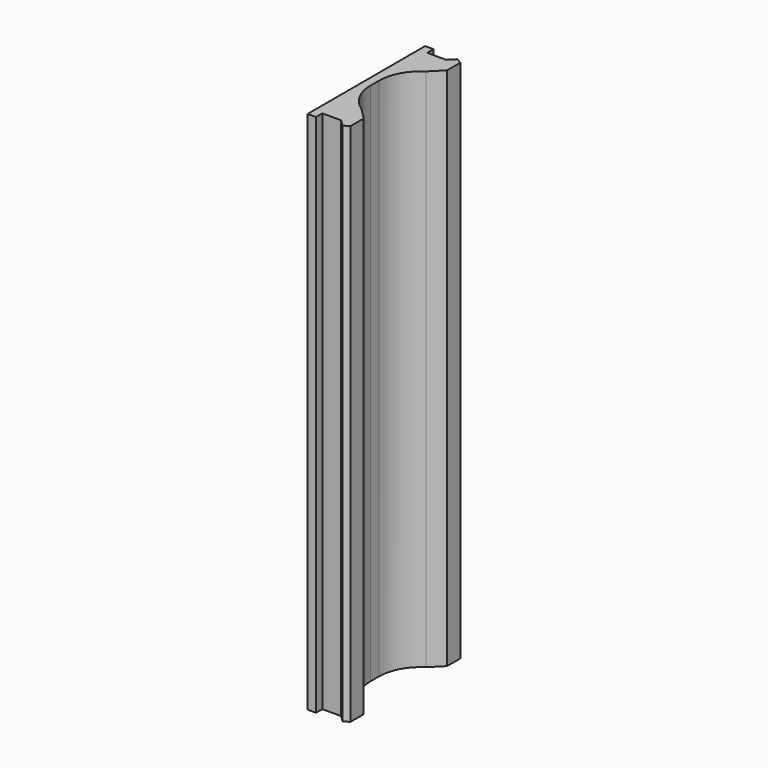
from build123d import *

# Parameters (mm, degrees)
F1_DEPTH    = 25
F2_T1_DEPTH = 25


# Not quite as in the source:
# - a fillet or chamfer that OpenCascade refuses, or shapes differently, is made with other operations: its cross-section is extruded or revolved along the edge and cut away or added


with BuildPart() as f1:
    # F0 (on Top) → F1 (new body)
    with BuildSketch(Plane.XY):
        Polygon((-6.8274033331, 3.5), (-7.2274033331, 3.5), (-7.2274033331, 0), (-7.2274033331, -3.5), (-6.8274033331, -3.5), (-6.8274033331, -3.125), (-5.9274033331, -3.125), (-5.6274033331, -3.425), (-5.3675957119, -3.275), (-5.3675957119, -2.4848076211), (-5.9274033331, -1.925), (-6.8274033331, -1.925), (-6.8274033331, -0.6), (-6.8274033331, 0.6), (-6.8274033331, 1.925), (-5.9274033331, 1.925), (-5.3675957119, 2.4848076211), (-5.3675957119, 3.275), (-5.6274033331, 3.425), (-5.9274033331, 3.125), (-6.8274033331, 3.125), align=None)
    extrude(amount=F1_DEPTH)

    # F2: fillet of radius 2 on 2 edges, made by hand

    # F2_s2 → F2_t1 (join)
    with BuildSketch(Plane.XY):
        with BuildLine():
            ThreePointArc((-5.9274033331, 1.925), (-6.5880850192, 1.2033539892), (-6.8274033331, 0.2546706911))
            Line((-6.8274033331, 0.2546706911), (-6.8274033331, 1.925))
            Line((-6.8274033331, 1.925), (-5.9274033331, 1.925))
        make_face()
        with BuildLine():
            ThreePointArc((-6.8274033331, -0.2546706911), (-6.5880850192, -1.2033539892), (-5.9274033331, -1.925))
            Line((-5.9274033331, -1.925), (-6.8274033331, -1.925))
            Line((-6.8274033331, -1.925), (-6.8274033331, -0.2546706911))
        make_face()
    extrude(amount=F2_T1_DEPTH)


solid = f1.part
